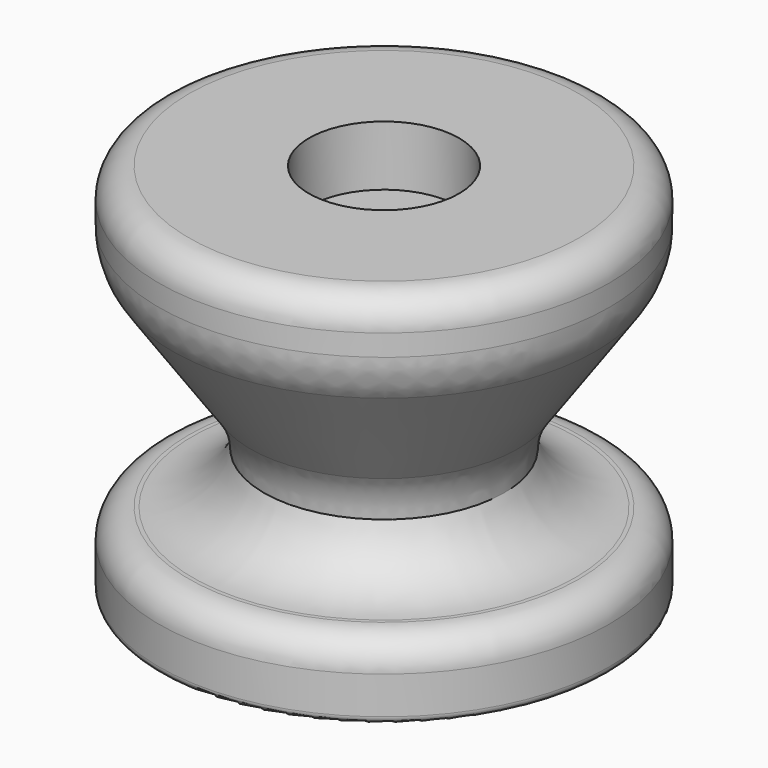
from build123d import *

# Parameters (mm, degrees)
F2_R           = 5
F4_R           = 2.5
F5_DEPTH       = 25.001
F6_D           = 5
F6_CBORE_D     = 10
F6_CBORE_DEPTH = 4


# Not quite as in the source:
# - a fillet or chamfer that OpenCascade refuses, or shapes differently, is made with other operations: its cross-section is extruded or revolved along the edge and cut away or added


with BuildPart() as f1:
    # F0 (on Front) → F1 (revolve)
    with BuildSketch(Plane.XZ):
        with BuildLine():
            Line((0, 25), (0, 0))
            Line((0, 0), (14.5, 0))
            ThreePointArc((14.5, 0), (14.8535533906, 0.1464466094), (15, 0.5))
            Line((15, 0.5), (15, 3))
            ThreePointArc((15, 3), (14.4142135624, 4.4142135624), (13, 5))
            Line((13, 5), (8, 5))
            Line((8, 5), (8, 10))
            Line((8, 10), (15, 20))
            Line((15, 20), (15, 23))
            ThreePointArc((15, 23), (14.4142135624, 24.4142135624), (13, 25))
            Line((13, 25), (0, 25))
        make_face()
    revolve(axis=Axis((0, 0, 12.5), (0, 0, -1)))

    # F2
    f2_edges = [f1.edges().sort_by_distance(p)[0] for p in [
        (-8, 0, 10),
        (-15, 0, 20),
        (11.5, 0, 15),
    ]]
    fillet(f2_edges, radius=F2_R)

    # F3: fillet of radius 5 on 3 edges, made by hand

    # F3_s1 → F3_t2 (revolve)
    with BuildSketch(Plane.XZ):
        with BuildLine():
            ThreePointArc((7.9999979579, 8.4238888459), (9.8193871029, 5.9453387459), (12.7450873806, 5))
            Line((12.7450873806, 5), (8, 5))
            Line((8, 5), (7.9999979579, 8.4238888459))
        make_face()
    revolve(axis=Axis((0, 0, 5), (0, 0, -1)))

    # F4 (on face) → F5 (cut, through all)
    with BuildSketch(Plane.XY.offset(25)):
        Circle(F4_R)
    extrude(amount=-F5_DEPTH, mode=Mode.SUBTRACT)

    # F6 (through all)
    with Locations(Plane.XY.offset(25)):
        with Locations((0, 0)):
            CounterBoreHole(F6_D / 2, F6_CBORE_D / 2, F6_CBORE_DEPTH)


solid = f1.part
